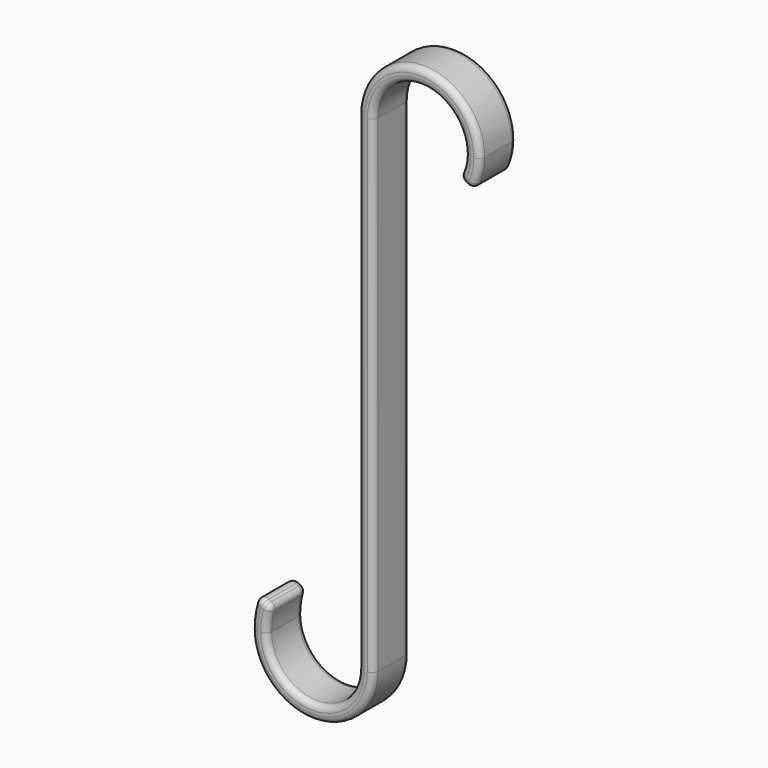
from build123d import *

# Parameters (mm, degrees)
F1_DEPTH = 19.05
F2_R     = 2.54


# Not quite as in the source:
# - a feature names something its author has since deleted; it is built from what else it names


with BuildPart() as f1:
    # F0 (on Front) → F1 (new body)
    with BuildSketch(Plane.XZ):
        with BuildLine():
            ThreePointArc((25.4, 0), (0, 25.4), (-25.4, 0))
            Line((-25.4, 0), (-25.4, -203.2))
            ThreePointArc((-25.4, -203.2), (-44.45, -222.25), (-63.5, -203.2))
            ThreePointArc((-63.5, -203.2), (-63.0744281022, -198.1179462529), (-61.8095664242, -193.177449652))
            Line((-61.8095664242, -193.177449652), (-67.3088277382, -190.002449652))
            ThreePointArc((-67.3088277382, -190.002449652), (-69.208925247, -196.4800131761), (-69.85, -203.2))
            ThreePointArc((-69.85, -203.2), (-44.45, -228.6), (-19.05, -203.2))
            Line((-19.05, -203.2), (-19.05, 0))
            ThreePointArc((-19.05, 0), (4.9305028092, 18.4008869908), (16.4977839421, -9.525))
            Line((16.4977839421, -9.525), (21.9970452561, -12.7))
            ThreePointArc((21.9970452561, -12.7), (24.5345159877, -6.5740037456), (25.4, 0))
        make_face()
    extrude(amount=F1_DEPTH)

    # F2
    f2_edges = [f1.edges().sort_by_distance(p)[0] for p in [
        (-61.809566, -9.525, -193.17745),
        (-67.308828, -9.525, -190.00245),
        (-64.559197, 0, -191.58995),
        (-64.559197, -19.05, -191.58995),
        (16.497784, -9.525, -9.525),
        (21.997045, -9.525, -12.7),
        (19.247415, 0, -11.1125),
        (19.247415, -19.05, -11.1125),
        (-19.05, 0, -101.6),
        (4.930503, 0, 18.400887),
        (6.574004, 0, 24.534516),
        (-25.4, 0, -101.6),
        (-44.45, 0, -222.25),
        (-63.074428, 0, -198.117946),
        (-69.208925, 0, -196.480013),
        (-44.45, 0, -228.6),
        (-19.05, -19.05, -101.6),
        (4.930503, -19.05, 18.400887),
        (6.574004, -19.05, 24.534516),
        (-25.4, -19.05, -101.6),
        (-44.45, -19.05, -222.25),
        (-63.074428, -19.05, -198.117946),
        (-69.208925, -19.05, -196.480013),
        (-44.45, -19.05, -228.6),
    ]]
    fillet(f2_edges, radius=F2_R)


solid = f1.part
